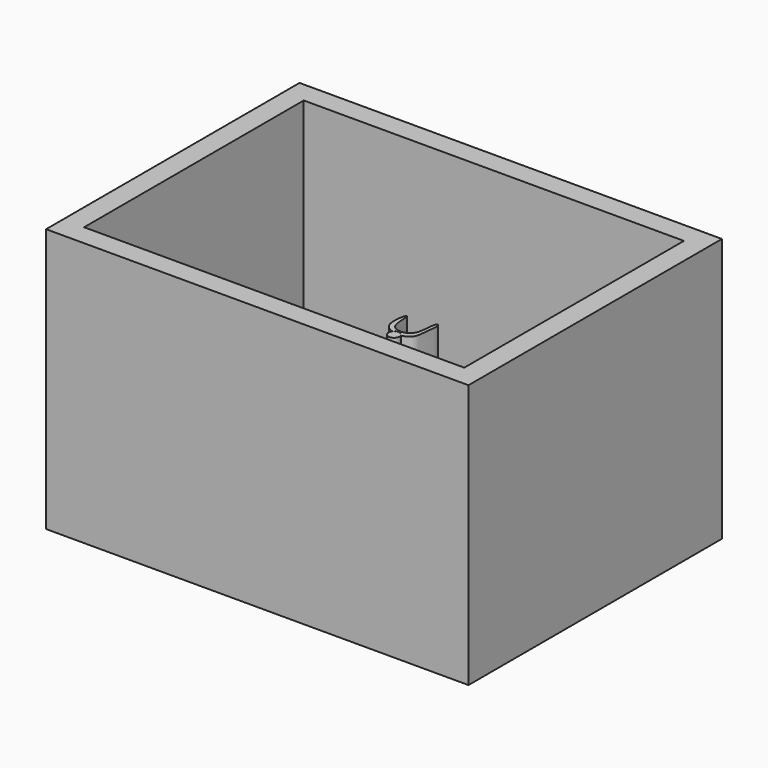
from build123d import *

# Parameters (mm, degrees)
F0_W      = 40
F0_H      = 30
F1_DEPTH  = 25
F2_T      = -2
F3_R      = 1.1734555852
F4_DEPTH  = 10
F5_R      = 1.1082567549
F6_DEPTH  = 10
F7_R      = 2.8596482252
F8_DEPTH  = 25
F12_R     = 1.9211371815
F13_DEPTH = 10
F19_DEPTH = 10
F21_DEPTH = 10
F23_DEPTH = 10
F25_DEPTH = 10
F27_DEPTH = 10
F29_DEPTH = 10
F31_DEPTH = 10
F34_DEPTH = 10
F36_DEPTH = 10
F38_DEPTH = 10
F40_DEPTH = 10
F42_R     = 0.5216317559
F43_DEPTH = 10
F45_DEPTH = 10
F47_R     = 0.3510274815
F48_DEPTH = 10
F50_DEPTH = 10
F53_DEPTH = 10
F57_DEPTH = 10
F59_R     = 0.5108467367
F60_DEPTH = 10
F62_R     = 0.3336573654
F63_DEPTH = 10
F64_R     = 0.3198907941
F65_DEPTH = 10
F67_DEPTH = 10
F69_DEPTH = 10
F72_DEPTH = 10


# Not quite as in the source:
# - a feature names something its author has since deleted; it is built from what else it names
# - the program builds the solid bodies; features that only make, move or delete a surface that nothing else refers to are left out


with BuildPart() as f1:
    # F0 (on Top) → F1 (new body)
    with BuildSketch(Plane.XY):
        with Locations((20, 15)):
            Rectangle(F0_W, F0_H)
    extrude(amount=F1_DEPTH)

    # F2
    f2_openings = [f1.faces().sort_by_distance(p)[0] for p in [
        (20, 15, 25),
    ]]
    offset(amount=F2_T, openings=f2_openings)


with BuildPart() as f4:
    # F3 (on face) → F4 (new body)
    with BuildSketch(Plane.XY.offset(2)):
        with Locations((33.0649241805, 17.3798706383)):
            Circle(F3_R)
    extrude(amount=F4_DEPTH)


with BuildPart() as f6:
    # F5 (on face) → F6 (new body)
    with BuildSketch(Plane.XY.offset(2)):
        with Locations((34.2975892127, 13.8197271153)):
            Circle(F5_R)
    extrude(amount=F6_DEPTH)


with BuildPart() as f8:
    # F7 (on face) → F8 (new body)
    with BuildSketch(Plane.XY.offset(2)):
        with Locations((21.9554807991, 20.8907555789)):
            Circle(F7_R)
    extrude(amount=F8_DEPTH)


with BuildPart() as f13:
    # F12 (on face) → F13 (new body)
    with BuildSketch(Plane.XY.offset(2)):
        with Locations((32.9036824405, 15)):
            Circle(F12_R)
    extrude(amount=F13_DEPTH)


with BuildPart() as f19:
    # F18 (on face) → F19 (new body)
    with BuildSketch(Plane.XY.offset(2)):
        with BuildLine():
            add(Edge.make_bspline(
                [(31.1595872045, 16.4146274328), (31.3460777814, 16.441681508), (31.6791584322, 19.3220044998), (28.384653062, 20.4572781756), (24.6426224505, 22.0539548755), (27.8703939641, 19.7801363072), (29.4048219075, 19.1897428524), (30.598723504, 18.2152304286), (30.9946239483, 16.390696313), (31.1595872045, 16.4146274328)],
                knots=[0, 0, 0, 0, 0.1392146887, 0.3254512731, 0.473844966, 0.6219230789, 0.7555027667, 0.8768553954, 1, 1, 1, 1], degree=3))
        make_face()
    extrude(amount=F19_DEPTH)


with BuildPart() as f21:
    # F20 (on face) → F21 (new body)
    with BuildSketch(Plane.XY.offset(2)):
        with BuildLine():
            add(Edge.make_bspline(
                [(33.1699363887, 17.5969358534), (33.4076153463, 17.9358086079), (33.5153282795, 18.7922089064), (31.5434469438, 21.3059142679), (32.8699232879, 18.6886341915), (32.437192172, 17.9259857829), (32.4337624015, 16.9000614182), (32.9890060839, 17.3389729633), (33.1699363887, 17.5969358534)],
                knots=[0, 0, 0, 0, 0.1754265945, 0.3872970316, 0.5846548671, 0.744659741, 0.8664585727, 1, 1, 1, 1], degree=3))
        make_face()
    extrude(amount=F21_DEPTH)


with BuildPart() as f23:
    # F22 (on face) → F23 (new body)
    with BuildSketch(Plane.XY.offset(2)):
        with BuildLine():
            add(Edge.make_bspline(
                [(30.3411670029, 15.4399722815), (30.2009584172, 15.8379624515), (29.9700974484, 16.570344431), (30.0810568548, 17.8366611028), (28.2138156632, 18.8999824626), (26.4468349348, 17.8309214555), (24.0819422893, 19.070255527), (25.6341742725, 17.2741910806), (27.1781032678, 17.7386953155), (28.9841492252, 17.9581919625), (29.5614246607, 16.5817369164), (29.6231261221, 14.8111577693), (30.6947775876, 14.4838796045), (30.4544604792, 15.1183822043), (30.3411670029, 15.4399722815)],
                knots=[0, 0, 0, 0, 0.0782358202, 0.1544987991, 0.2484756097, 0.3526906555, 0.4424157453, 0.5224285132, 0.6154464448, 0.7056158792, 0.7871760731, 0.8817812698, 0.9367827013, 1, 1, 1, 1], degree=3))
        make_face()
    extrude(amount=F23_DEPTH)


with BuildPart() as f25:
    # F24 (on face) → F25 (new body)
    with BuildSketch(Plane.XY.offset(2)):
        with BuildLine():
            add(Edge.make_bspline(
                [(30.4293595254, 13.6394565925), (29.9274874741, 13.0877413673), (26.9587408771, 12.5246699265), (22.6562615975, 17.8390597065), (26.7368241926, 14.3117481695), (28.264728778, 13.5590201873), (29.9463011451, 14.0047073219), (30.7408465197, 14.4729517561), (30.6515057919, 13.8836652052), (30.4293595254, 13.6394565925)],
                knots=[0, 0, 0, 0, 0.184379902, 0.390024994, 0.5650471983, 0.7099284611, 0.839769227, 0.918386954, 1, 1, 1, 1], degree=3))
        make_face()
    extrude(amount=F25_DEPTH)


with BuildPart() as f27:
    # F26 (on face) → F27 (new body)
    with BuildSketch(Plane.XY.offset(2)):
        with BuildLine():
            add(Edge.make_bspline(
                [(31.2069114298, 12.9553740844), (30.8637240181, 12.870849006), (28.4359577194, 9.4632607274), (27.0032096593, 14.4323225338), (22.7292757543, 10.3426112937), (26.7618426369, 13.5633268171), (28.2703725846, 8.9337677225), (31.1518711195, 11.6773182122), (31.4024955111, 13.0035453146), (31.2069114298, 12.9553740844)],
                knots=[0, 0, 0, 0, 0.156556993, 0.3098269175, 0.4601868427, 0.5955673381, 0.7553278537, 0.910777451, 1, 1, 1, 1], degree=3))
        make_face()
    extrude(amount=F27_DEPTH)


with BuildPart() as f29:
    # F28 (on face) → F29 (new body)
    with BuildSketch(Plane.XY.offset(2)):
        with BuildLine():
            add(Edge.make_bspline(
                [(32.7289775014, 12.2271766886), (32.628121124, 12.2945738034), (31.4546133417, 9.1759520365), (28.1423760284, 9.3827454945), (26.8988796942, 8.6704019519), (29.9774325304, 8.7628337308), (32.1547342752, 9.0576112716), (32.8291078679, 12.1602647294), (32.7289775014, 12.2271766886)],
                knots=[0, 0, 0, 0, 0.181579815, 0.388195544, 0.475048613, 0.6440064242, 0.8197272805, 1, 1, 1, 1], degree=3))
        make_face()
    extrude(amount=F29_DEPTH)


with BuildPart() as f31:
    # F30 (on face) → F31 (new body)
    with BuildSketch(Plane.XY.offset(2)):
        with BuildLine():
            add(Edge.make_bspline(
                [(34.0808182955, 11.7869656533), (34.2216314985, 11.8513348039), (35.4316398489, 11.0506302824), (33.0806820362, 7.7178065759), (34.4931879316, 10.5390414384), (33.9242725705, 11.7154047831), (34.0808182955, 11.7869656533)],
                knots=[0, 0, 0, 0, 0.203113003, 0.5116706097, 0.774193956, 1, 1, 1, 1], degree=3))
        make_face()
    extrude(amount=F31_DEPTH)


with BuildPart() as f34:
    # F33 (on face) → F34 (new body)
    with BuildSketch(Plane.XY.offset(2)):
        with BuildLine():
            ThreePointArc((24.7804066452, 21.6932493016), (25.2727212719, 21.6749981013), (25.5242986297, 22.0985729247))
            ThreePointArc((25.5242986297, 22.0985729247), (25.3830156941, 22.439660104), (25.0419285148, 22.5809430396))
            ThreePointArc((25.0419285148, 22.5809430396), (24.5792207613, 22.2348904311), (24.7804066452, 21.6932493016))
        make_face()
        with BuildLine():
            ThreePointArc((24.7804066452, 21.6932493016), (24.5792207613, 22.2348904311), (25.0419285148, 22.5809430396))
            add(Edge.make_bspline(
                [(24.7804066452, 21.6932493016), (24.747730564, 21.4033667543), (24.6604732744, 20.6278061665), (22.2133901733, 21.0046180316), (21.5754956832, 21.7201628788), (22.8987021583, 21.4634593716), (24.0287316408, 21.333274223), (23.9570056337, 22.1499701098), (24.4487301076, 22.9485041462), (23.8604704661, 23.8798406026), (23.8311898384, 24.7763731956), (24.699650061, 24.0280313363), (24.9139209062, 23.1221271374), (25.0419285148, 22.5809430396)],
                knots=[0, 0, 0, 0, 0.0833598511, 0.22313493, 0.2893530308, 0.3838020122, 0.4778048106, 0.549862148, 0.6366549002, 0.7342728908, 0.8032689451, 0.882482578, 1, 1, 1, 1], degree=3))
        make_face()
    extrude(amount=F34_DEPTH)


with BuildPart() as f36:
    # F35 (on face) → F36 (new body)
    with BuildSketch(Plane.XY.offset(2)):
        with BuildLine():
            ThreePointArc((23.7088892609, 18.1679258034), (24.0751086339, 18.3196188345), (24.2268016651, 18.6858382076))
            ThreePointArc((24.2268016651, 18.6858382076), (23.9082791676, 19.1638308054), (23.3445021809, 19.0538807518))
            ThreePointArc((23.3445021809, 19.0538807518), (23.2299074985, 18.4888363555), (23.7088892609, 18.1679258034))
        make_face()
        with BuildLine():
            ThreePointArc((23.7088892609, 18.1679258034), (23.2299074985, 18.4888363555), (23.3445021809, 19.0538807518))
            add(Edge.make_bspline(
                [(23.7088892609, 18.1679258034), (23.5761690549, 17.8857829166), (23.2737412381, 17.2428676429), (20.2673059027, 16.6568939273), (22.6649117703, 17.7668092291), (22.967695978, 18.0667088003), (22.6638322676, 18.7084395997), (22.9051948901, 19.4349054452), (22.1401452945, 20.1627144722), (21.8610684961, 20.622605655), (22.6095105141, 20.617031609), (23.2055186347, 19.8498458305), (23.1817036062, 19.4912390376), (23.2879025299, 19.2058772701), (23.3445021809, 19.0538807518)],
                knots=[0, 0, 0, 0, 0.0994249826, 0.2265610498, 0.3450525525, 0.4091193579, 0.4828732125, 0.5637329989, 0.6609396868, 0.7173452518, 0.7859127947, 0.878687087, 0.9353936202, 1, 1, 1, 1], degree=3))
        make_face()
    extrude(amount=F36_DEPTH)


with BuildPart() as f38:
    # F37 (on face) → F38 (new body)
    with BuildSketch(Plane.XY.offset(2)):
        with BuildLine():
            ThreePointArc((23.1239311397, 15.1295968465), (23.4789716382, 15.2766594361), (23.6260342278, 15.6316999346))
            ThreePointArc((23.6260342278, 15.6316999346), (23.4198023489, 16.0373694289), (22.9705204796, 16.1097926876))
            ThreePointArc((22.9705204796, 16.1097926876), (22.7482752008, 15.9648517418), (22.6309315736, 15.7268783928))
            add(Edge.make_bspline(
                [(22.6309315736, 15.7268783928), (22.6802317795, 15.646400148), (22.6861919564, 15.54721642), (22.6630457306, 15.4324710441)],
                knots=[0.5352845212, 0.5352845212, 0.5352845212, 0.5352845212, 0.5744626895, 0.5744626895, 0.5744626895, 0.5744626895], degree=3))
            ThreePointArc((22.6630457306, 15.4324710441), (22.8481830029, 15.2120924083), (23.1239311397, 15.1295968465))
        make_face()
        with BuildLine():
            ThreePointArc((22.6309315736, 15.7268783928), (22.7482752008, 15.9648517418), (22.9705204796, 16.1097926876))
            add(Edge.make_bspline(
                [(22.9705204796, 16.1097926876), (22.760760095, 16.2496048638), (22.2565708633, 16.5849880829), (20.5506728599, 16.2876293852), (20.2617734725, 15.4380113495), (21.4221602566, 16.1090672395), (22.4806463634, 15.9722057643), (22.6309315736, 15.7268783928)],
                knots=[0, 0, 0, 0, 0.0984249405, 0.2365850006, 0.3066971304, 0.4158550145, 0.5352845212, 0.5352845212, 0.5352845212, 0.5352845212], degree=3))
        make_face()
        with BuildLine():
            add(Edge.make_bspline(
                [(22.6630457306, 15.4324710441), (22.6162783719, 15.2006259819), (22.2005070042, 14.4590012134), (21.5378604008, 12.9320722787), (22.9906220707, 14.0604546364), (23.0789588636, 14.7689549605), (23.1239311397, 15.1295968465)],
                knots=[0.5744626895, 0.5744626895, 0.5744626895, 0.5744626895, 0.653622872, 0.7732170873, 0.8845697866, 1, 1, 1, 1], degree=3))
            ThreePointArc((23.1239311397, 15.1295968465), (22.8481830029, 15.2120924083), (22.6630457306, 15.4324710441))
        make_face()
        with BuildLine():
            add(Edge.make_bspline(
                [(22.6309315736, 15.7268783928), (22.6802317795, 15.646400148), (22.6861919564, 15.54721642), (22.6630457306, 15.4324710441)],
                knots=[0.5352845212, 0.5352845212, 0.5352845212, 0.5352845212, 0.5744626895, 0.5744626895, 0.5744626895, 0.5744626895], degree=3))
            ThreePointArc((22.6309315736, 15.7268783928), (22.6247888171, 15.5772531451), (22.6630457306, 15.4324710441))
        make_face()
    extrude(amount=F38_DEPTH)


with BuildPart() as f40:
    # F39 (on face) → F40 (new body)
    with BuildSketch(Plane.XY.offset(2)):
        with BuildLine():
            ThreePointArc((23.7906227456, 10.696652594), (23.8309428709, 10.7880998629), (23.8447329783, 10.8870854601))
            ThreePointArc((23.8447329783, 10.8870854601), (23.5320112052, 11.245850933), (23.1339178415, 10.9850267668))
            ThreePointArc((23.1339178415, 10.9850267668), (23.3369677322, 10.5554923286), (23.7906227456, 10.696652594))
        make_face()
        with BuildLine():
            ThreePointArc((23.7906227456, 10.696652594), (23.3369677322, 10.5554923286), (23.1339178415, 10.9850267668))
            add(Edge.make_bspline(
                [(23.7906227456, 10.696652594), (24.2110580294, 10.3297704812), (25.0573682314, 9.5910451599), (23.6428733469, 7.2787588204), (24.0857373105, 8.8556648528), (24.2227103572, 9.5916799076), (23.3706918708, 10.2474373954), (22.623131789, 10.8418523738), (21.462450855, 10.5697381266), (20.6394698869, 10.7804611716), (22.1091845713, 11.129932844), (22.7867792047, 11.0341312171), (23.1339178415, 10.9850267668)],
                knots=[0, 0, 0, 0, 0.1231836231, 0.2480593639, 0.3390609539, 0.4276782317, 0.5241770294, 0.6197159009, 0.7287036968, 0.7923235414, 0.893624236, 1, 1, 1, 1], degree=3))
        make_face()
    extrude(amount=F40_DEPTH)


with BuildPart() as f43:
    # F42 (on face) → F43 (new body)
    with BuildSketch(Plane.XY.offset(2)):
        with Locations((24.9590612948, 22.3981905729)):
            Circle(F42_R)
    extrude(amount=F43_DEPTH)


with BuildPart() as f45:
    # F44 (on face) → F45 (new body)
    with BuildSketch(Plane.XY.offset(2)):
        with BuildLine():
            add(Edge.make_bspline(
                [(25.3651738167, 22.7433908731), (25.5114259921, 22.7109935356), (26.247088781, 23.1500558234), (26.3760792355, 24.0833631327), (26.2806745456, 25.0041518456), (26.0039307584, 25.5781394445), (25.9579644767, 24.1727179481), (25.7947258871, 23.2738551316), (24.6780489825, 22.9230133977), (23.7635728507, 23.5856924699), (23.7144375222, 24.706584579), (23.5808441807, 25.8222578935), (23.201967471, 25.5244422074), (23.4690808082, 24.0517849403), (23.4789632894, 22.9222936006), (24.4884002954, 22.51931354), (24.4948161568, 22.6753760996), (24.6229536661, 22.8145023121), (24.7903671423, 22.9308990834), (25.0067947355, 22.9463642635), (25.2480942451, 22.9102536009), (25.2941518545, 22.7591234423), (25.3651738167, 22.7433908731)],
                knots=[0, 0, 0, 0, 0.0581371888, 0.1211561532, 0.1848406612, 0.2189506354, 0.2847134755, 0.3478038611, 0.4104878932, 0.4731951552, 0.5433887389, 0.6041891688, 0.6324950179, 0.7098849246, 0.7798723973, 0.8372785929, 0.8554652824, 0.8829079513, 0.9118011697, 0.9415966991, 0.9717678235, 1, 1, 1, 1], degree=3))
        make_face()
    extrude(amount=F45_DEPTH)


with BuildPart() as f48:
    # F47 (on face) → F48 (new body)
    with BuildSketch(Plane.XY.offset(2)):
        with Locations((24.1662617773, 18.9750436693)):
            Circle(F47_R)
    extrude(amount=F48_DEPTH)


with BuildPart() as f50:
    # F49 (on face) → F50 (new body)
    with BuildSketch(Plane.XY.offset(2)):
        with BuildLine():
            add(Edge.make_bspline(
                [(23.8155461848, 18.8523400575), (23.833950912, 18.8610158591), (23.76764463, 19.0457253719), (23.8557475286, 19.1829525404), (24.0123172201, 19.3455535764), (24.226641487, 19.3240649886), (24.678119978, 19.4311821862), (24.8675021214, 20.2436971713), (24.8481083527, 20.7351098184), (24.7672193983, 21.2809926497), (24.5143394632, 20.7554536343), (24.6144239289, 19.9418836531), (24.0331707486, 19.5394350099), (23.0534781898, 19.6251104746), (22.7255694376, 20.5380724496), (22.6072693229, 20.97076614), (22.4274917234, 20.6635148282), (22.7575464968, 19.8203682245), (23.3648957317, 19.1373796665), (23.576981743, 19.0913518206), (23.7915215016, 18.8410150657), (23.8155461848, 18.8523400575)],
                knots=[0, 0, 0, 0, 0.0325094602, 0.0655318885, 0.101068993, 0.1366875416, 0.1864967681, 0.2555677125, 0.3159294386, 0.361528975, 0.4081761551, 0.4799280147, 0.5410248023, 0.6140055245, 0.690793982, 0.7345559139, 0.7678092676, 0.8437485108, 0.9182991956, 0.9575636481, 1, 1, 1, 1], degree=3))
        make_face()
    extrude(amount=F50_DEPTH)


with BuildPart() as f53:
    # F52 (on face) → F53 (new body)
    with BuildSketch(Plane.XY.offset(2)):
        with BuildLine():
            add(Edge.make_bspline(
                [(24.0386221558, 19.3411465734), (24.1040984928, 19.3713043604), (24.2673018769, 19.3502502565), (25.0932319554, 19.4679121943), (24.8629354384, 20.7618071215), (24.2595021441, 21.7724369487), (24.5824102589, 20.3199226655), (24.7312352656, 19.8208344603), (23.7593875301, 19.6171597369), (22.856274225, 19.9330686729), (22.5505608995, 21.0801820944), (21.696821224, 21.0762245838), (22.7947637004, 19.8562080132), (23.3527401827, 19.3984058222), (23.8023149238, 19.1381724078), (23.9687629131, 19.3089700612), (24.0386221558, 19.3411465734)],
                knots=[0, 0, 0, 0, 0.0414625498, 0.1089636894, 0.2048269873, 0.273976187, 0.3609921763, 0.4202460503, 0.4971121447, 0.5800054603, 0.6698075991, 0.7218442443, 0.8189478623, 0.9000916462, 0.955761998, 1, 1, 1, 1], degree=3))
        make_face()
    extrude(amount=F53_DEPTH)


with BuildPart() as f57:
    # F56 (on face) → F57 (new body)
    with BuildSketch(Plane.XY.offset(2)):
        with BuildLine():
            add(Edge.make_bspline(
                [(23.779662326, 19.0007314086), (23.776310863, 18.9247837857), (23.867899625, 18.7954509155), (23.625166884, 18.4408937739), (23.0552566853, 17.7242940261), (20.9236074862, 18.0108238037), (22.1335279505, 18.1945343847), (22.974348048, 18.2042050885), (23.4436627349, 18.9380532029), (23.8598892119, 20.012424989), (22.4429790292, 21.5592113966), (23.5956187481, 21.0297287711), (24.0051809774, 19.9352009104), (24.0904128395, 19.4047294157), (24.0603444403, 19.3375666069), (23.9049459402, 19.3118003918), (23.7839271018, 19.097375646), (23.779662326, 19.0007314086)],
                knots=[0, 0, 0, 0, 0.0377750836, 0.0881071014, 0.1706250725, 0.2717332239, 0.3371742484, 0.4175840731, 0.4915792622, 0.5818318817, 0.6819084231, 0.7474804345, 0.8438221175, 0.9021917138, 0.9206130483, 0.9519307648, 1, 1, 1, 1], degree=3))
        make_face()
    extrude(amount=F57_DEPTH)


with BuildPart() as f60:
    # F59 (on face) → F60 (new body)
    with BuildSketch(Plane.XY.offset(2)):
        with Locations((23.1938697398, 15.8582534641)):
            Circle(F59_R)
    extrude(amount=F60_DEPTH)


with BuildPart() as f63:
    # F62 (on face) → F63 (new body)
    with BuildSketch(Plane.XY.offset(2)):
        with Locations((23.536330089, 16.3223296404)):
            Circle(F62_R)
    extrude(amount=F63_DEPTH)


with BuildPart() as f65:
    # F64 (on face) → F65 (new body)
    with BuildSketch(Plane.XY.offset(2)):
        with Locations((23.6197020859, 11.0648004338)):
            Circle(F64_R)
    extrude(amount=F65_DEPTH)


with BuildPart() as f67:
    # F66 (on face) → F67 (new body)
    with BuildSketch(Plane.XY.offset(2)):
        with BuildLine():
            add(Edge.make_bspline(
                [(21.5124003589, 16.8080888689), (21.4975874788, 16.882536345), (22.1503945533, 17.1985239599), (23.2290671268, 17.3114278341), (23.3416791933, 16.5784572322), (23.2228269914, 16.5119448085), (23.1358210654, 16.3344607007), (23.3050154789, 16.0844634713), (23.387428011, 15.5062212064), (22.5004948486, 14.8299977434), (21.789948531, 14.4148063299), (22.4678079453, 15.3022923221), (23.0441230836, 15.6293949474), (22.9160422995, 16.5121427337), (22.9327015569, 16.9668631112), (22.1158395091, 16.712729008), (21.5259782634, 16.7398482085), (21.5124003589, 16.8080888689)],
                knots=[0, 0, 0, 0, 0.073806303, 0.1655644278, 0.2306760243, 0.261394134, 0.2975053344, 0.3451022304, 0.4087851862, 0.5063824691, 0.5669901467, 0.6449717623, 0.7208342164, 0.8022777278, 0.8524925312, 0.9323470571, 1, 1, 1, 1], degree=3))
        make_face()
    extrude(amount=F67_DEPTH)


with BuildPart() as f69:
    # F68 (on face) → F69 (new body)
    with BuildSketch(Plane.XY.offset(2)):
        with BuildLine():
            add(Edge.make_bspline(
                [(20.9286995232, 12.0301982388), (20.9710833612, 12.2353374694), (22.3783879172, 12.5046868919), (23.3448709495, 12.88744255), (23.6569103797, 11.5549239747), (23.3000813931, 11.3696048788), (23.2561581879, 11.0840380346), (23.3714846182, 10.7048545544), (23.7665156839, 10.8337612174), (24.4657975613, 10.0899241918), (22.7828082287, 7.4164856485), (23.198209513, 9.2028656986), (23.5538310098, 9.9563158405), (22.7511659215, 10.9677240757), (22.9520867729, 12.219241452), (21.6859955271, 11.4881630212), (20.8979075119, 11.8811638469), (20.9286995232, 12.0301982388)],
                knots=[0, 0, 0, 0, 0.0891250087, 0.1609587332, 0.2349236956, 0.2771079472, 0.3152309913, 0.3567531573, 0.3974416442, 0.4628259421, 0.5698914403, 0.6391338764, 0.7096229117, 0.7905253372, 0.8575134669, 0.9352503593, 1, 1, 1, 1], degree=3))
        make_face()
    extrude(amount=F69_DEPTH)


with BuildPart() as f72:
    # F71 (on face) → F72 (new body)
    with BuildSketch(Plane.XY.offset(2)):
        with BuildLine():
            add(Edge.make_bspline(
                [(21.3742181659, 11.8522271514), (21.4093748699, 11.966088385), (22.4383820183, 12.0949612901), (23.3771307091, 11.5146016726), (23.3679778646, 11.2934011114), (23.296264729, 11.2108917842), (23.2644079892, 10.9707354071), (23.491421019, 10.6904327777), (23.8687872702, 10.87199934), (24.2305770639, 10.0713521327), (22.933327197, 8.047239016), (23.2109136356, 9.1213031918), (23.7479188693, 10.0189453426), (23.1268816449, 10.6482658553), (23.0468233183, 11.3603737174), (22.2755970329, 11.633756444), (21.6620529032, 11.5923889996), (21.3547378862, 11.7891368039), (21.3742181659, 11.8522271514)],
                knots=[0, 0, 0, 0, 0.0819766737, 0.1688189159, 0.2005254825, 0.2265539652, 0.2657462974, 0.3109559948, 0.3555584302, 0.4246191147, 0.5349913627, 0.5928427731, 0.6778976231, 0.7495825952, 0.8163907322, 0.8866381043, 0.9545768418, 1, 1, 1, 1], degree=3))
        make_face()
    extrude(amount=F72_DEPTH)


with BuildPart() as f73_1:
    # F73: instance of F13
    add(f13.part.mirror(Plane.YZ.offset(20)))


with BuildPart() as f73_2:
    # F73: instance of F19
    add(f19.part.mirror(Plane.YZ.offset(20)))


with BuildPart() as f73_3:
    # F73: instance of F21
    add(f21.part.mirror(Plane.YZ.offset(20)))


with BuildPart() as f73_4:
    # F73: instance of F27
    add(f27.part.mirror(Plane.YZ.offset(20)))


with BuildPart() as f73_5:
    # F73: instance of F29
    add(f29.part.mirror(Plane.YZ.offset(20)))


with BuildPart() as f73_6:
    # F73: instance of F25
    add(f25.part.mirror(Plane.YZ.offset(20)))


with BuildPart() as f73_7:
    # F73: instance of F23
    add(f23.part.mirror(Plane.YZ.offset(20)))


with BuildPart() as f73_8:
    # F73: instance of F31
    add(f31.part.mirror(Plane.YZ.offset(20)))


with BuildPart() as f73_9:
    # F73: instance of F43
    add(f43.part.mirror(Plane.YZ.offset(20)))


with BuildPart() as f73_10:
    # F73: instance of F45
    add(f45.part.mirror(Plane.YZ.offset(20)))


with BuildPart() as f73_11:
    # F73: instance of F48
    add(f48.part.mirror(Plane.YZ.offset(20)))


with BuildPart() as f73_12:
    # F73: instance of F57
    add(f57.part.mirror(Plane.YZ.offset(20)))


with BuildPart() as f73_13:
    # F73: instance of F63
    add(f63.part.mirror(Plane.YZ.offset(20)))


with BuildPart() as f73_14:
    # F73: instance of F65
    add(f65.part.mirror(Plane.YZ.offset(20)))


with BuildPart() as f73_15:
    # F73: instance of F67
    add(f67.part.mirror(Plane.YZ.offset(20)))


with BuildPart() as f73_16:
    # F73: instance of F72
    add(f72.part.mirror(Plane.YZ.offset(20)))


solid = Compound([f1.part, f13.part, f19.part, f21.part, f23.part, f25.part, f27.part, f29.part, f31.part, f43.part, f45.part, f48.part, f57.part, f63.part, f65.part, f67.part, f72.part, f73_1.part, f73_2.part, f73_3.part, f73_4.part, f73_5.part, f73_6.part, f73_7.part, f73_8.part, f73_9.part, f73_10.part, f73_11.part, f73_12.part, f73_13.part, f73_14.part, f73_15.part, f73_16.part])
